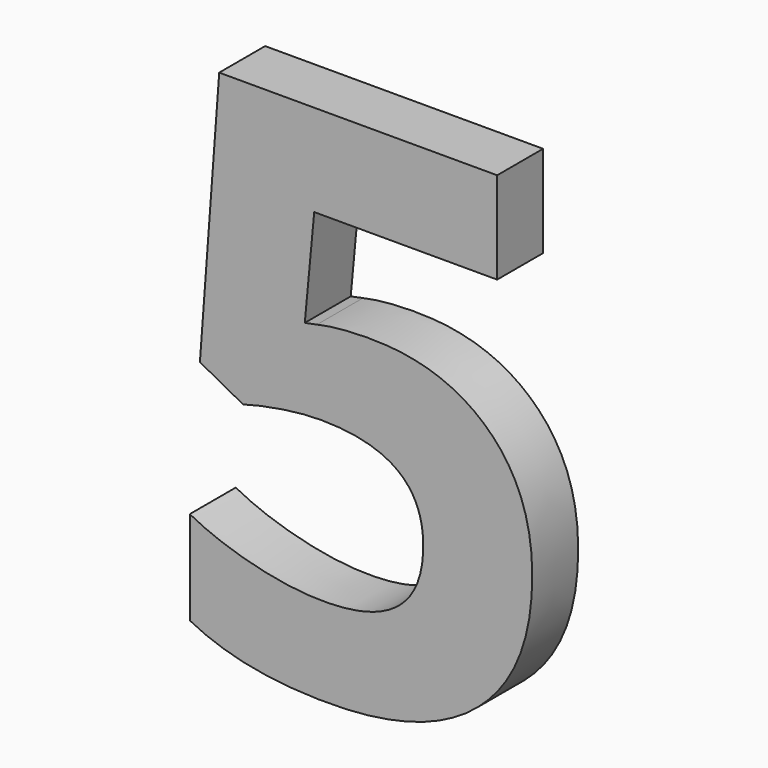
from build123d import *

# Parameters (mm, degrees)
F0_TEXT_SIZE = 62.5
F1_DEPTH     = 5


# Not quite as in the source:
# - Text() gives the source's letters only with a copy of the font that has no kerning and outlines rounded to 1/6400 em; it was checked with that copy


with BuildPart() as f1:
    # F0 (on Front) → F1 (new body)
    with BuildSketch(Plane.XZ):
        with Locations((-66.4385901389, 20.0860716127)):
            Text('5', F0_TEXT_SIZE, font='Open Sans', font_style=FontStyle.BOLD, text_align=(TextAlign.LEFT, TextAlign.BOTTOM))
    extrude(amount=F1_DEPTH)


solid = f1.part
